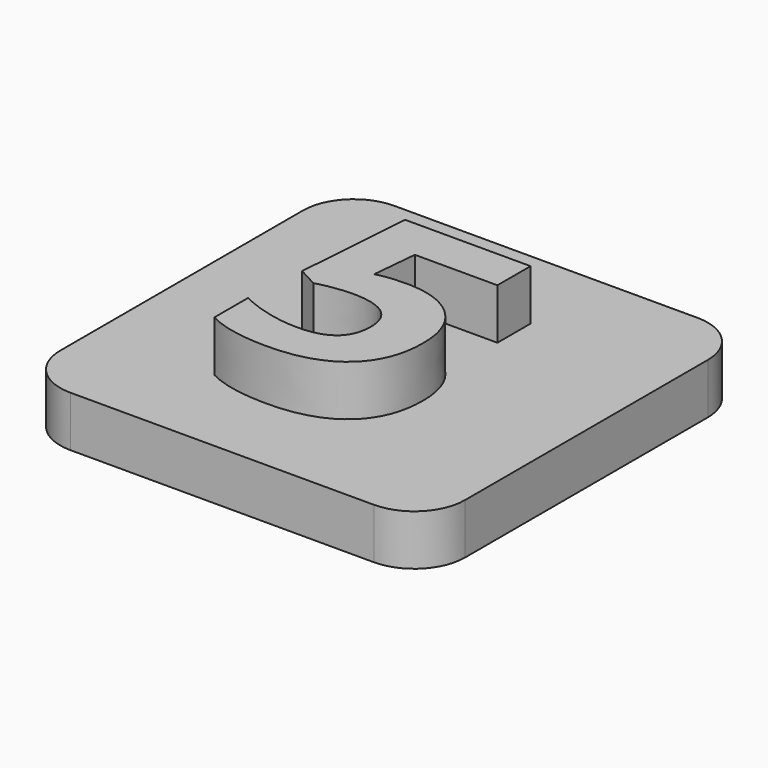
from build123d import *

# Parameters (mm, degrees)
F1_DEPTH     = 6.35
F2_TEXT_SIZE = 40.6554913045
F3_DEPTH     = 6.35


# Not quite as in the source:
# - Text() gives the source's letters only with a copy of the font that has no kerning and outlines rounded to 1/6400 em; it was checked with that copy


with BuildPart() as f1:
    # F0 (on Top) → F1 (new body)
    with BuildSketch(Plane.XY):
        with BuildLine():
            Line((-12.3437797487, 56.3756098591), (-50.4437797487, 56.3756098591))
            ThreePointArc((-50.4437797487, 56.3756098591), (-54.9339078092, 54.5157379196), (-56.7937797487, 50.0256098591))
            Line((-56.7937797487, 50.0256098591), (-56.7937797487, 11.9256098591))
            ThreePointArc((-56.7937797487, 11.9256098591), (-54.9339078092, 7.4354817985), (-50.4437797487, 5.5756098591))
            Line((-50.4437797487, 5.5756098591), (-12.3437797487, 5.5756098591))
            ThreePointArc((-12.3437797487, 5.5756098591), (-7.8536516881, 7.4354817985), (-5.9937797487, 11.9256098591))
            Line((-5.9937797487, 11.9256098591), (-5.9937797487, 50.0256098591))
            ThreePointArc((-5.9937797487, 50.0256098591), (-7.8536516881, 54.5157379196), (-12.3437797487, 56.3756098591))
        make_face()
    extrude(amount=F1_DEPTH)

    # F2 (on face) → F3 (join)
    with BuildSketch(Plane.XY.offset(6.35)):
        with Locations((-43.7685344368, 16.1692658439)):
            Text('5', F2_TEXT_SIZE, font='Open Sans', font_style=FontStyle.BOLD, text_align=(TextAlign.LEFT, TextAlign.BOTTOM))
    extrude(amount=F3_DEPTH)


solid = f1.part
